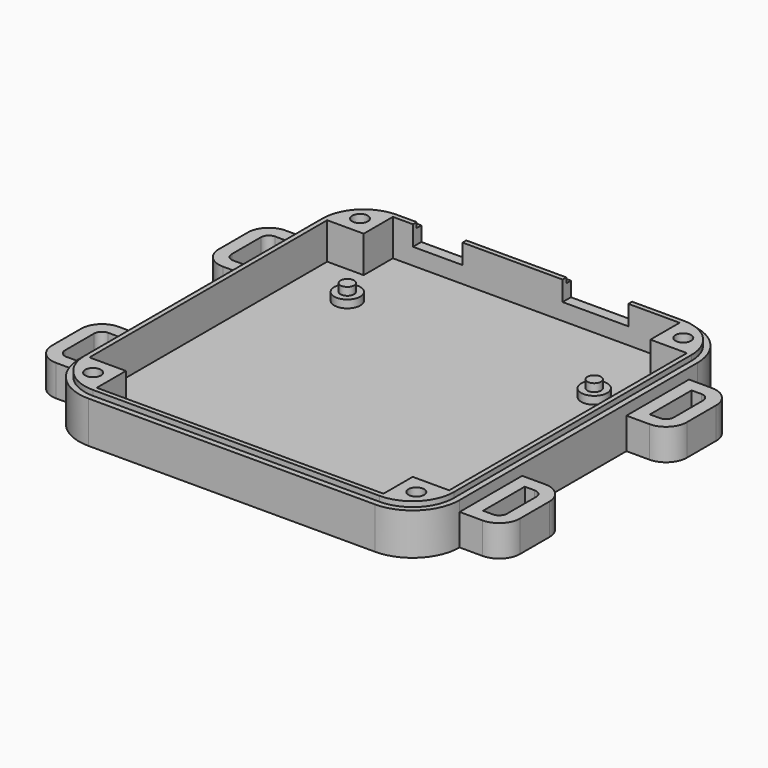
from build123d import *

# Parameters (mm, degrees)
F1_DEPTH  = 2
F2_DEPTH  = 6
F3_R      = 2.5
F4_DEPTH  = 1.5
F5_R      = 1.3
F6_DEPTH  = 1.5
F8_DEPTH  = 7
F9_R      = 1.5
F10_DEPTH = 10
F11_W     = 12.6
F11_H     = 2
F11_W_2   = 9.5
F12_DEPTH = 3.8
F13_R     = 3
F14_DEPTH = 0.4
F15_SIZE  = 1.49999
F16_W     = 19.2
F16_H     = 1.1
F17_DEPTH = 1


# Not quite as in the source:
# - a fillet or chamfer is up to 0.001 mm smaller than in the source, because OpenCascade refuses the exact size


with BuildPart() as f1:
    # F0 (on Top) → F1 (new body)
    with BuildSketch(Plane.XY):
        with BuildLine():
            Line((27.5, 38.5), (-27.5, 38.5))
            ThreePointArc((-27.5, 38.5), (-33.8639610307, 35.8639610307), (-36.5, 29.5))
            Line((-36.5, 29.5), (-36.5, 27.5))
            Line((-36.5, 27.5), (-36.5, 12.5))
            Line((-36.5, 12.5), (-36.5, -12.5))
            Line((-36.5, -12.5), (-36.5, -27.5))
            ThreePointArc((-36.5, -27.5), (-33.8639610307, -33.8639610307), (-27.5, -36.5))
            Line((-27.5, -36.5), (27.5, -36.5))
            ThreePointArc((27.5, -36.5), (33.8639610307, -33.8639610307), (36.5, -27.5))
            Line((36.5, -27.5), (36.5, -12.5))
            Line((36.5, -12.5), (36.5, 12.5))
            Line((36.5, 12.5), (36.5, 27.5))
            Line((36.5, 27.5), (36.5, 29.5))
            ThreePointArc((36.5, 29.5), (33.8639610307, 35.8639610307), (27.5, 38.5))
        make_face()
    extrude(amount=F1_DEPTH)

    # F0 (on Top) → F2 (join)
    with BuildSketch(Plane.XY):
        with BuildLine():
            Line((-36.5, 12.5), (-36.5, 27.5))
            Line((-36.5, 27.5), (-40.9, 27.5))
            ThreePointArc((-40.9, 27.5), (-43.7284271247, 26.3284271247), (-44.9, 23.5))
            Line((-44.9, 23.5), (-44.9, 16.5))
            ThreePointArc((-44.9, 16.5), (-43.7284271247, 13.6715728753), (-40.9, 12.5))
            Line((-40.9, 12.5), (-36.5, 12.5))
        make_face()
        with BuildLine():
            Line((-40.9, 25.0000007004), (-38.9999992996, 25.0000007004))
            Line((-38.9999992996, 25.0000007004), (-38.9999992996, 14.9999992996))
            Line((-38.9999992996, 14.9999992996), (-40.9, 14.9999992996))
            ThreePointArc((-40.9, 14.9999992996), (-41.960660667, 15.439339333), (-42.4000007004, 16.5))
            Line((-42.4000007004, 16.5), (-42.4000007004, 23.5))
            ThreePointArc((-42.4000007004, 23.5), (-41.960660667, 24.560660667), (-40.9, 25.0000007004))
        make_face(mode=Mode.SUBTRACT)
        with BuildLine():
            Line((-36.5, -27.5), (-36.5, -12.5))
            Line((-36.5, -12.5), (-40.9, -12.5))
            ThreePointArc((-40.9, -12.5), (-43.7284271247, -13.6715728753), (-44.9, -16.5))
            Line((-44.9, -16.5), (-44.9, -23.5))
            ThreePointArc((-44.9, -23.5), (-43.7284271247, -26.3284271247), (-40.9, -27.5))
            Line((-40.9, -27.5), (-36.5, -27.5))
        make_face()
        with BuildLine():
            Line((-38.9999992996, -14.9999992996), (-38.9999992996, -25.0000007004))
            Line((-38.9999992996, -25.0000007004), (-40.9, -25.0000007004))
            ThreePointArc((-40.9, -25.0000007004), (-41.960660667, -24.560660667), (-42.4000007004, -23.5))
            Line((-42.4000007004, -23.5), (-42.4000007004, -16.5))
            ThreePointArc((-42.4000007004, -16.5), (-41.960660667, -15.439339333), (-40.9, -14.9999992996))
            Line((-40.9, -14.9999992996), (-38.9999992996, -14.9999992996))
        make_face(mode=Mode.SUBTRACT)
        with BuildLine():
            Line((40.9, 27.5), (36.5, 27.5))
            Line((36.5, 27.5), (36.5, 12.5))
            Line((36.5, 12.5), (40.9, 12.5))
            ThreePointArc((40.9, 12.5), (43.7284271247, 13.6715728753), (44.9, 16.5))
            Line((44.9, 16.5), (44.9, 23.5))
            ThreePointArc((44.9, 23.5), (43.7284271247, 26.3284271247), (40.9, 27.5))
        make_face()
        with BuildLine():
            Line((40.9, 14.9999992996), (38.9999992996, 14.9999992996))
            Line((38.9999992996, 14.9999992996), (38.9999992996, 25.0000007004))
            Line((38.9999992996, 25.0000007004), (40.9, 25.0000007004))
            ThreePointArc((40.9, 25.0000007004), (41.960660667, 24.560660667), (42.4000007004, 23.5))
            Line((42.4000007004, 23.5), (42.4000007004, 16.5))
            ThreePointArc((42.4000007004, 16.5), (41.960660667, 15.439339333), (40.9, 14.9999992996))
        make_face(mode=Mode.SUBTRACT)
        with BuildLine():
            Line((40.9, -12.5), (36.5, -12.5))
            Line((36.5, -12.5), (36.5, -27.5))
            Line((36.5, -27.5), (40.9, -27.5))
            ThreePointArc((40.9, -27.5), (43.7284271247, -26.3284271247), (44.9, -23.5))
            Line((44.9, -23.5), (44.9, -16.5))
            ThreePointArc((44.9, -16.5), (43.7284271247, -13.6715728753), (40.9, -12.5))
        make_face()
        with BuildLine():
            Line((38.9999992996, -14.9999992996), (40.9, -14.9999992996))
            ThreePointArc((40.9, -14.9999992996), (41.960660667, -15.439339333), (42.4000007004, -16.5))
            Line((42.4000007004, -16.5), (42.4000007004, -23.5))
            ThreePointArc((42.4000007004, -23.5), (41.960660667, -24.560660667), (40.9, -25.0000007004))
            Line((40.9, -25.0000007004), (38.9999992996, -25.0000007004))
            Line((38.9999992996, -25.0000007004), (38.9999992996, -14.9999992996))
        make_face(mode=Mode.SUBTRACT)
    extrude(amount=F2_DEPTH)

    # F3 (on face) → F4 (join)
    with BuildSketch(Plane.XY.offset(2)):
        with Locations((-18.94, -30.6)):
            Circle(F3_R)
        with Locations((8.96, -30.6)):
            Circle(F3_R)
        with Locations((24.16, 20.2)):
            Circle(F3_R)
        with Locations((-24.24, 21.5)):
            Circle(F3_R)
    extrude(amount=F4_DEPTH)

    # F5 (on face) → F6 (join)
    with BuildSketch(Plane.XY.offset(3.5)):
        with Locations((-19.24, -30.6)):
            Circle(F5_R)
        with Locations((8.96, -30.6)):
            Circle(F5_R)
        with Locations((24.16, 20.2)):
            Circle(F5_R)
        with Locations((-24.24, 21.5)):
            Circle(F5_R)
    extrude(amount=F6_DEPTH)

    # F7 (on face) → F8 (join)
    with BuildSketch(Plane.XY.offset(2)):
        with BuildLine():
            Line((27.5, 38.5), (-27.5, 38.5))
            ThreePointArc((-27.5, 38.5), (-33.8639610307, 35.8639610307), (-36.5, 29.5))
            Line((-36.5, 29.5), (-36.5, -27.5))
            ThreePointArc((-36.5, -27.5), (-33.8639610307, -33.8639610307), (-27.5, -36.5))
            Line((-27.5, -36.5), (27.5, -36.5))
            ThreePointArc((27.5, -36.5), (33.8639610307, -33.8639610307), (36.5, -27.5))
            Line((36.5, -27.5), (36.5, 29.5))
            ThreePointArc((36.5, 29.5), (33.8639610307, 35.8639610307), (27.5, 38.5))
        make_face()
        Polygon((-27.5, 29.5), (-27.5, 36.5), (27.5, 36.5), (27.5, 29.5), (34.5, 29.5), (34.5, -27.5), (27.5, -27.5), (27.5, -34.5), (-27.5, -34.5), (-27.5, -27.5), (-34.5, -27.5), (-34.5, 29.5), align=None, mode=Mode.SUBTRACT)
    extrude(amount=F8_DEPTH)

    # F9 (on face) → F10 (cut)
    with BuildSketch(Plane.XY.offset(9)):
        with Locations((-31, 33)):
            Circle(F9_R)
        with Locations((31, 33)):
            Circle(F9_R)
        with Locations((-31, -31)):
            Circle(F9_R)
        with Locations((31, -31)):
            Circle(F9_R)
    extrude(amount=-F10_DEPTH, mode=Mode.SUBTRACT)

    # F11 (on face) → F12 (cut)
    with BuildSketch(Plane.XY.offset(9)):
        with Locations((11.36, 37.5)):
            Rectangle(F11_W, F11_H)
        with Locations((-18.89, 37.5)):
            Rectangle(F11_W_2, F11_H)
    extrude(amount=-F12_DEPTH, mode=Mode.SUBTRACT)

    # F13 (on face) → F14 (cut)
    with BuildSketch(Plane(origin=(0, 0, 0), x_dir=(1, 0, 0), z_dir=(0, 0, -1))):
        with Locations((31, -33)):
            Circle(F13_R)
        with Locations((-31, -33)):
            Circle(F13_R)
        with Locations((-31, 31)):
            Circle(F13_R)
        with Locations((31, 31)):
            Circle(F13_R)
    extrude(amount=-F14_DEPTH, mode=Mode.SUBTRACT)

    # F15 (size 1.5 in the source; OpenCascade refuses exactly that, so slightly less here)
    f15_edges = [f1.edges().sort_by_distance(p)[0] for p in [
        (29.5, 33, 0.4),
        (-32.5, 33, 0.4),
        (29.5, -31, 0.4),
        (-32.5, -31, 0.4),
    ]]
    chamfer(f15_edges, length=F15_SIZE)

    # F16 (on face) → F17 (cut)
    with BuildSketch(Plane.XY.offset(9)):
        with BuildLine():
            Line((-23.64, 38.5), (-27.5, 38.5))
            ThreePointArc((-27.5, 38.5), (-33.8639610307, 35.8639610307), (-36.5, 29.5))
            Line((-36.5, 29.5), (-36.5, -27.5))
            ThreePointArc((-36.5, -27.5), (-33.8639610307, -33.8639610307), (-27.5, -36.5))
            Line((-27.5, -36.5), (27.5, -36.5))
            ThreePointArc((27.5, -36.5), (33.8639610307, -33.8639610307), (36.5, -27.5))
            Line((36.5, -27.5), (36.5, 29.5))
            ThreePointArc((36.5, 29.5), (33.8639610307, 35.8639610307), (27.5, 38.5))
            Line((27.5, 38.5), (17.66, 38.5))
            Line((17.66, 38.5), (17.66, 37.4))
            Line((17.66, 37.4), (27.5, 37.4))
            ThreePointArc((27.5, 37.4), (33.0861435714, 35.0861435714), (35.4, 29.5))
            Line((35.4, 29.5), (35.4, -27.5))
            ThreePointArc((35.4, -27.5), (33.0861435714, -33.0861435714), (27.5, -35.4))
            Line((27.5, -35.4), (-27.5, -35.4))
            ThreePointArc((-27.5, -35.4), (-33.0861435714, -33.0861435714), (-35.4, -27.5))
            Line((-35.4, -27.5), (-35.4, 29.5))
            ThreePointArc((-35.4, 29.5), (-33.0861435714, 35.0861435714), (-27.5, 37.4))
            Line((-27.5, 37.4), (-23.64, 37.4))
            Line((-23.64, 37.4), (-23.64, 38.5))
        make_face()
        with Locations((-4.54, 37.95)):
            Rectangle(F16_W, F16_H)
    extrude(amount=-F17_DEPTH, mode=Mode.SUBTRACT)


solid = f1.part
